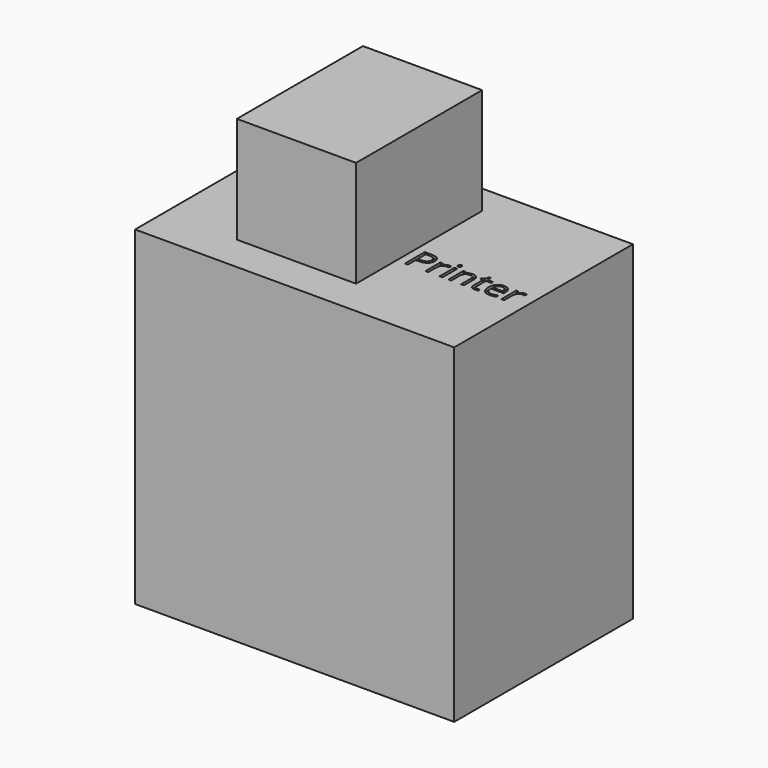
from build123d import *

# Parameters (mm, degrees)
F0_W         = 762
F0_H         = 533.4
F1_DEPTH     = 787.4
F2_W         = 284.6163511276
F2_H         = 376.2395307422
F3_DEPTH     = 254
F4_TEXT_SIZE = 82.8690826893
F5_DEPTH     = 6.35


# Not quite as in the source:
# - a length typed as a fraction of an inch, garbled in the dataset ("3 / 203.2 mm" for 3/8 in), is restored
# - Text() gives the source's letters only with a copy of the font that has no kerning and outlines rounded to 1/6400 em; it was checked with that copy


with BuildPart() as f1:
    # F0 (on Top) → F1 (new body)
    with BuildSketch(Plane.XY):
        with Locations((381, 266.7)):
            Rectangle(F0_W, F0_H)
    extrude(amount=F1_DEPTH)

    # F2 (on face) → F3 (join)
    with BuildSketch(Plane.XY.offset(787.4)):
        with Locations((316.2322044373, 274.5309211314)):
            Rectangle(F2_W, F2_H)
    extrude(amount=F3_DEPTH)

    # F4 (on face) → F5 (cut)
    with BuildSketch(Plane.XY.offset(787.4)):
        with Locations((470.7251191139, 207.0342604637)):
            Text('Printer', F4_TEXT_SIZE, font='Open Sans', text_align=(TextAlign.LEFT, TextAlign.BOTTOM))
    extrude(amount=-F5_DEPTH, mode=Mode.SUBTRACT)


solid = f1.part
